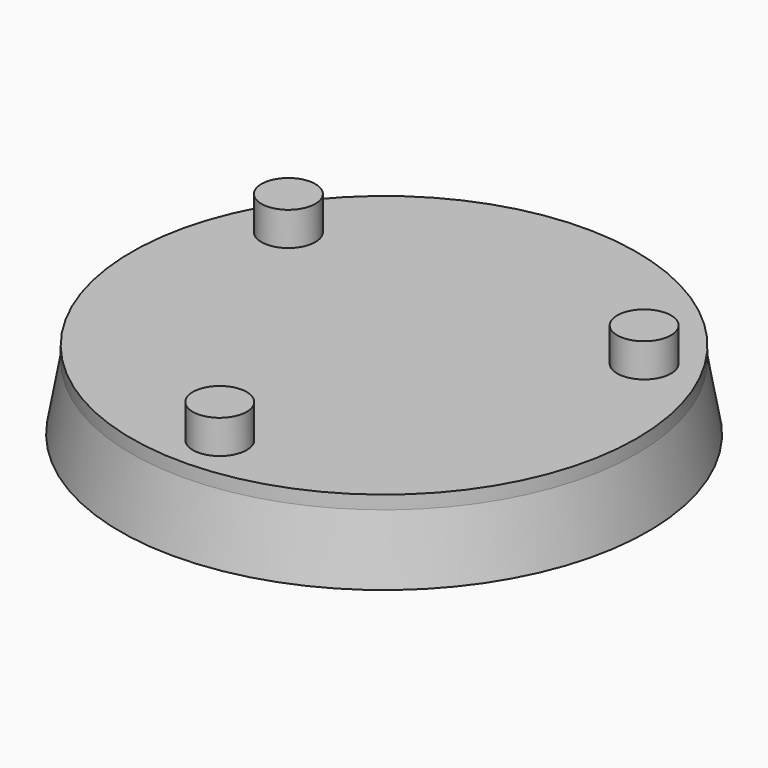
from build123d import *

# Parameters (mm, degrees)
F3_R             = 37.5
F4_DEPTH         = 2
F8_R             = 4
F9_DEPTH         = 5
F7_R             = 2.5
F10_DEPTH        = 5
F10_TAPER        = 2
F14_COPIES_COUNT = 2
F16_COPIES_COUNT = 2


# Not quite as in the source:
# - a pattern or mirror of a feature is missing from the dataset's text; its kind, count and spacing are read off the source's solid


with BuildPart() as f2:
    # F1 (on Front) → F2 (revolve)
    with BuildSketch(Plane.XZ):
        with BuildLine():
            Line((-16, 0), (-21.33, 0))
            ThreePointArc((-21.33, 0), (-18.665, -2.665), (-16, 0))
        make_face()
    revolve(axis=Axis((0, 0, 18.396249041), (0, 0, 1)))

    # F3 (on face) → F4 (join)
    with BuildSketch(Plane.XY):
        Circle(F3_R)
    extrude(amount=F4_DEPTH)

    # F5 (on Right) → F6 (revolve)
    with BuildSketch(Plane.YZ):
        Polygon((-36.8366060944, -9.6), (-35.1438670796, 0), (-37.5, 0), (-39.1927390148, -9.6), align=None)
    revolve(axis=Axis((0, 0, 18.396249041), (0, 0, 1)))

    # F8 (on face) → F9 (join)
    with BuildSketch(Plane.XY.offset(2)):
        with Locations((0, -30.5)):
            Circle(F8_R)
        with Locations((26.4137748154, 15.25)):
            Circle(F8_R)
        with Locations((-26.4137748154, 15.25)):
            Circle(F8_R)
    extrude(amount=F9_DEPTH)

    # F7 (on face) → F10 (cut)
    with BuildSketch(Plane(origin=(0, 0, 0), x_dir=(1, 0, 0), z_dir=(0, 0, -1))):
        with Locations((0, 30.5)):
            Circle(F7_R)
        with Locations((-26.4137748154, -15.25)):
            Circle(F7_R)
        with Locations((26.4137748154, -15.25)):
            Circle(F7_R)
    extrude(amount=-F10_DEPTH, taper=F10_TAPER, mode=Mode.SUBTRACT)

    # F13 (on offset) → F14 (join, up to the next surface of F2)
    with BuildSketch(Plane.YZ.offset(33)):
        with BuildLine():
            Line((2.5, 0), (-2.5, 0))
            ThreePointArc((-2.5, 0), (0, -2.5), (2.5, 0))
        make_face()
    f14 = extrude(until=Until.NEXT)

    # F14_copies: F14 ×2 about axis
    f14_copies_axis = Axis((0, 0, 0), (0, 0, 1))
    for i in range(1, F14_COPIES_COUNT):
        add(f14.rotate(f14_copies_axis, i * 360 / F14_COPIES_COUNT))

    # F15 (on offset) → F16 (join, up to the next surface of F2)
    with BuildSketch(Plane.YZ.offset(23)):
        with BuildLine():
            Line((1, 0), (-1, 0))
            ThreePointArc((-1, 0), (0, -1), (1, 0))
        make_face()
    f16 = extrude(until=Until.NEXT, dir=(-1, 0, 0))

    # F16_copies: F16 ×2 about axis
    f16_copies_axis = Axis((0, 0, 0), (0, 0, 1))
    for i in range(1, F16_COPIES_COUNT):
        add(f16.rotate(f16_copies_axis, i * 360 / F16_COPIES_COUNT))

    # F16_face (on face) → F17 section 0
    with BuildSketch(Plane(origin=(23, 0, -0.4244131816), x_dir=(0, 1, 0), z_dir=(1, 0, 0))):
        with BuildLine():
            Line((1, 0.4244131816), (-1, 0.4244131816))
            ThreePointArc((-1, 0.4244131816), (0, -0.5755868184), (1, 0.4244131816))
        make_face()
    # F14_face (on face) → F17 section 1
    with BuildSketch(Plane(origin=(33, 0, -1.0610329539), x_dir=(0, 1, 0), z_dir=(-1, 0, 0))):
        with BuildLine():
            Line((-2.5, -1.0610329539), (2.5, -1.0610329539))
            ThreePointArc((2.5, -1.0610329539), (0, 1.4389670461), (-2.5, -1.0610329539))
        make_face()
    f17 = loft()

    # F17_copies: F17 across plane
    add(f17.mirror(Plane(origin=(0, 0, 0), x_dir=(0, 0, -1), z_dir=(-1, 0, 0))))


solid = f2.part
